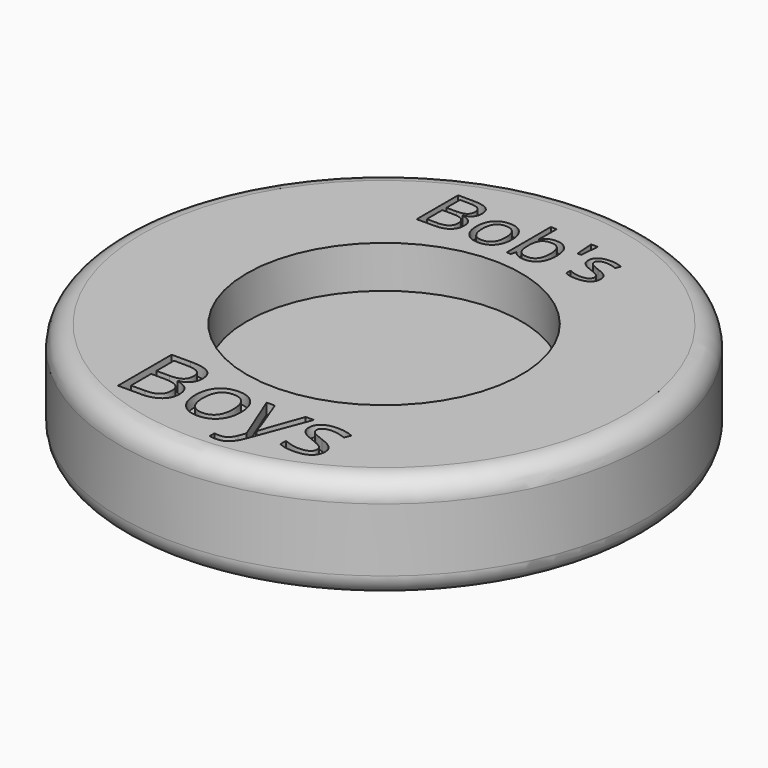
from build123d import *

# Parameters (mm, degrees)
F0_R           = 25
F1_DEPTH       = 10
F2_R           = 2
F4_D           = 26
F5_R           = 13
F6_DEPTH       = 6
F7_TEXT_SIZE   = 6.8746494233
F7_TEXT_SIZE_2 = 8.8967486388
F8_DEPTH       = 1


# Not quite as in the source:
# - Text() gives the source's letters only with a copy of the font that has no kerning and outlines rounded to 1/6400 em; it was checked with that copy


with BuildPart() as f1:
    # F0 (on Top) → F1 (new body)
    with BuildSketch(Plane.XY):
        Circle(F0_R)
    extrude(amount=F1_DEPTH)

    # F2
    f2_edges = [f1.edges().sort_by_distance(p)[0] for p in [
        (-25, 0, 10),
        (-25, 0, 0),
    ]]
    fillet(f2_edges, radius=F2_R)

    # F4 (through all)
    with Locations(Plane.XY.offset(10)):
        with Locations((0, 0)):
            Hole(F4_D / 2)

    # F5 (on face) → F6 (join)
    with BuildSketch(Plane(origin=(0, 0, 0), x_dir=(1, 0, 0), z_dir=(0, 0, -1))):
        Circle(F5_R)
    extrude(amount=-F6_DEPTH)

    # F7 (on face) → F8 (cut)
    with BuildSketch(Plane.XY.offset(10)):
        with Locations((-9.2783013824, 14.6126765758)):
            Text("Bob's", F7_TEXT_SIZE, font='Open Sans', text_align=(TextAlign.LEFT, TextAlign.BOTTOM))
        with Locations((-10.070757533, -20.0094329193)):
            Text('Boys', F7_TEXT_SIZE_2, font='Open Sans', text_align=(TextAlign.LEFT, TextAlign.BOTTOM))
    extrude(amount=-F8_DEPTH, mode=Mode.SUBTRACT)


solid = f1.part
